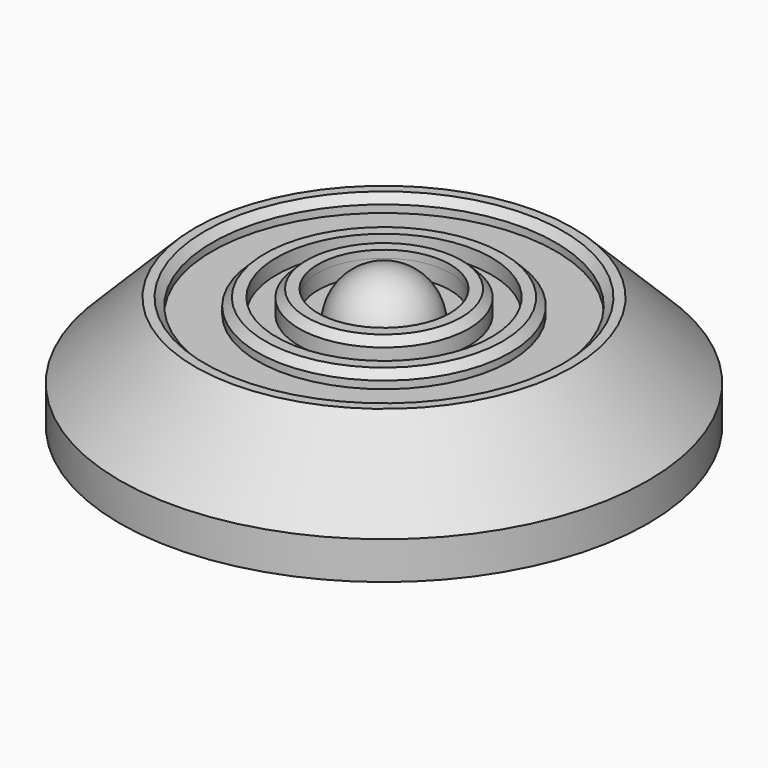
from build123d import *

# Parameters (mm, degrees)
F0_R         = 35
F1_DEPTH     = 15
F2_SIZE      = 10
F4_R         = 22.75
F4_R_2       = 16.75
F5_DEPTH     = 2
F4_R_3       = 14.25
F4_R_4       = 11.25
F6_DEPTH     = 2
F4_R_5       = 8.75
F7_DEPTH     = 2
F8_DEPTH     = 1
F12_R        = 30
F13_DEPTH    = 9.5
F15_R        = 32.5
F16_DEPTH    = 5
F17_S5_R     = 32.5
F17_T6_DEPTH = 48


# Not quite as in the source:
# - a fillet or chamfer that OpenCascade refuses, or shapes differently, is made with other operations: its cross-section is extruded or revolved along the edge and cut away or added


with BuildPart() as f1:
    # F0 (on Top) → F1 (new body)
    with BuildSketch(Plane.XY):
        Circle(F0_R)
    extrude(amount=F1_DEPTH)

    # F2
    f2_edges = [f1.edges().sort_by_distance(p)[0] for p in [
        (-35, 0, 15),
    ]]
    chamfer(f2_edges, length=F2_SIZE)

    # F4 (on offset) → F5 (cut)
    with BuildSketch(Plane.XY.offset(15)):
        Circle(F4_R)
        Circle(F4_R_2, mode=Mode.SUBTRACT)
    extrude(amount=-F5_DEPTH, mode=Mode.SUBTRACT)

    # F4 (on offset) → F6 (cut)
    with BuildSketch(Plane.XY.offset(15)):
        Circle(F4_R_3)
        Circle(F4_R_4, mode=Mode.SUBTRACT)
    extrude(amount=-F6_DEPTH, mode=Mode.SUBTRACT)

    # F4 (on offset) → F7 (cut)
    with BuildSketch(Plane.XY.offset(15)):
        Circle(F4_R_5)
    extrude(amount=-F7_DEPTH, mode=Mode.SUBTRACT)

    # F4 (on offset) → F8 (join)
    with BuildSketch(Plane.XY.offset(15)):
        Circle(F4_R_4)
        Circle(F4_R_5, mode=Mode.SUBTRACT)
    extrude(amount=F8_DEPTH)

    # F9 (on Front) → F10 (revolve)
    with BuildSketch(Plane.XZ):
        with BuildLine():
            Line((0, 12), (0, 5.5))
            ThreePointArc((0, 5.5), (4.5961940777, 7.4038059223), (6.5, 12))
            Line((6.5, 12), (0, 12))
        make_face()
        with BuildLine():
            Line((0, 18.5), (0, 12))
            Line((0, 12), (6.5, 12))
            ThreePointArc((6.5, 12), (4.5961940777, 16.5961940777), (0, 18.5))
        make_face()
    revolve(axis=Axis((0, 0, 6), (0, 0, 1)))

    # F11: chamfer of 1 on 3 edges, made by hand

    # F11_s1 → F11_t2 (revolve, cut)
    with BuildSketch(Plane.XZ):
        Polygon((23.75, 15), (22.75, 14), (22.75, 15), align=None)
    revolve(axis=Axis((0, 0, 15), (0, 0, 1)), mode=Mode.SUBTRACT)

    # F11_s3 → F11_t4 (revolve, cut)
    with BuildSketch(Plane.XZ):
        Polygon((16.75, 14), (15.75, 15), (16.75, 15), align=None)
    revolve(axis=Axis((0, 0, 15), (0, 0, 1)), mode=Mode.SUBTRACT)

    # F11_s5 → F11_t6 (revolve, cut)
    with BuildSketch(Plane.XZ):
        Polygon((11.25, 15), (10.25, 16), (11.25, 16), align=None)
    revolve(axis=Axis((0, 0, 16), (0, 0, 1)), mode=Mode.SUBTRACT)

    # F12 (on Top) → F13 (cut)
    with BuildSketch(Plane.XY):
        Circle(F12_R)
    extrude(amount=F13_DEPTH, mode=Mode.SUBTRACT)

    # F15 (on offset) → F16 (cut)
    with BuildSketch(Plane.XY.offset(1)):
        Circle(F15_R)
    extrude(amount=F16_DEPTH, mode=Mode.SUBTRACT)

    # F17: chamfer of 3 on 1 edges, made by hand


with BuildPart() as f17_tool2:
    # F17_s3 → F17_t4 (revolve)
    with BuildSketch(Plane.XZ):
        Polygon((33, 6), (30, 9), (30, 6), align=None)
    revolve(axis=Axis((0, 0, 6), (0, 0, -1)))

    # F17_s5 → F17_t6 (intersect, symmetric)
    with BuildSketch(Plane.XY.offset(7.5)):
        Circle(F17_S5_R)
    extrude(amount=F17_T6_DEPTH, both=True, mode=Mode.INTERSECT)


with BuildPart() as f1_1:
    add(f1.part)

    # F17_t1: cut F17_tool2
    add(f17_tool2.part, mode=Mode.SUBTRACT)


solid = f1_1.part
